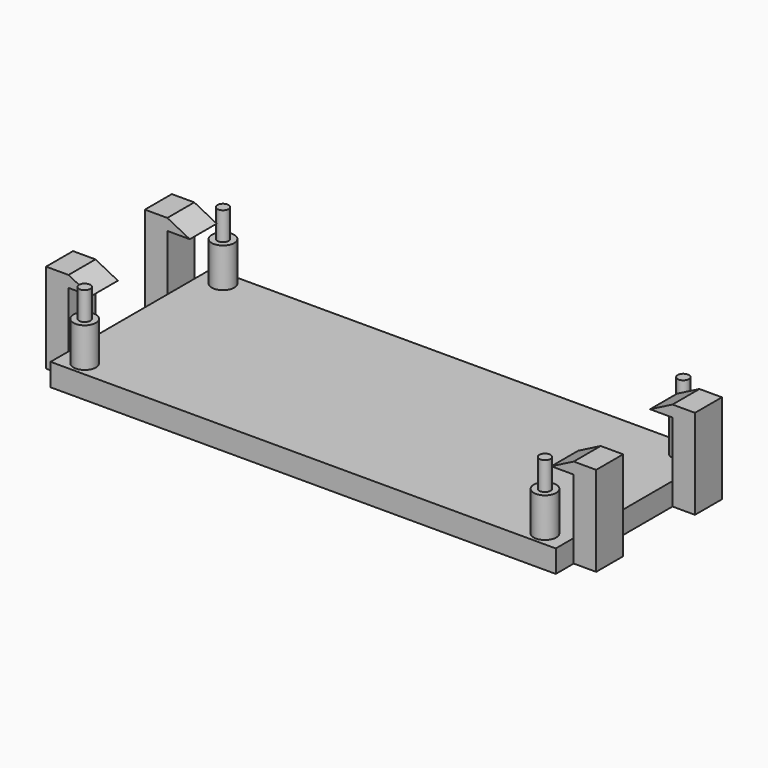
from build123d import *

# Parameters (mm, degrees)
F0_R     = 1
F0_R_2   = 0.5
F1_DEPTH = 2
F2_DEPTH = 5.5
F3_DEPTH = 8
F0_W     = 2
F0_H     = 3
F4_DEPTH = 8
F6_DEPTH = 3


# Not quite as in the source:
# - a feature names something its author has since deleted; it is built from what else it names


with BuildPart() as f1:
    # F0 (on Top) → F1 (new body)
    with BuildSketch(Plane.XY):
        Polygon((22.5, 9), (-22.5, 9), (-22.5, 7), (-22.5, 4), (-22.5, -4), (-22.5, -7), (-22.5, -9), (22.5, -9), (22.5, -7), (22.5, -4), (22.5, 4), (22.5, 7), align=None)
        with Locations((-20.5, -7.7)):
            Circle(F0_R, mode=Mode.SUBTRACT)
        with Locations((20.5, -7.7)):
            Circle(F0_R, mode=Mode.SUBTRACT)
        with Locations((-20.5, 7.7)):
            Circle(F0_R, mode=Mode.SUBTRACT)
        with Locations((20.5, 7.7)):
            Circle(F0_R, mode=Mode.SUBTRACT)
        with Locations((-20.5, 7.7)):
            Circle(F0_R)
        with Locations((-20.5, 7.7)):
            Circle(F0_R_2, mode=Mode.SUBTRACT)
        with Locations((20.5, 7.7)):
            Circle(F0_R)
        with Locations((20.5, 7.7)):
            Circle(F0_R_2, mode=Mode.SUBTRACT)
        with Locations((20.5, -7.7)):
            Circle(F0_R)
        with Locations((20.5, -7.7)):
            Circle(F0_R_2, mode=Mode.SUBTRACT)
        with Locations((-20.5, -7.7)):
            Circle(F0_R)
        with Locations((-20.5, -7.7)):
            Circle(F0_R_2, mode=Mode.SUBTRACT)
        with Locations((-20.5, 7.7)):
            Circle(F0_R_2)
        with Locations((20.5, 7.7)):
            Circle(F0_R_2)
        with Locations((20.5, -7.7)):
            Circle(F0_R_2)
        with Locations((-20.5, -7.7)):
            Circle(F0_R_2)
    extrude(amount=F1_DEPTH)

    # F0 (on Top) → F2 (join)
    with BuildSketch(Plane.XY):
        with Locations((-20.5, 7.7)):
            Circle(F0_R)
        with Locations((-20.5, 7.7)):
            Circle(F0_R_2, mode=Mode.SUBTRACT)
        with Locations((-20.5, 7.7)):
            Circle(F0_R_2)
        with Locations((-20.5, -7.7)):
            Circle(F0_R)
        with Locations((-20.5, -7.7)):
            Circle(F0_R_2, mode=Mode.SUBTRACT)
        with Locations((-20.5, -7.7)):
            Circle(F0_R_2)
        with Locations((20.5, 7.7)):
            Circle(F0_R)
        with Locations((20.5, 7.7)):
            Circle(F0_R_2, mode=Mode.SUBTRACT)
        with Locations((20.5, 7.7)):
            Circle(F0_R_2)
        with Locations((20.5, -7.7)):
            Circle(F0_R)
        with Locations((20.5, -7.7)):
            Circle(F0_R_2, mode=Mode.SUBTRACT)
        with Locations((20.5, -7.7)):
            Circle(F0_R_2)
    extrude(amount=F2_DEPTH)

    # F0 (on Top) → F3 (join)
    with BuildSketch(Plane.XY):
        with Locations((-20.5, 7.7)):
            Circle(F0_R_2)
        with Locations((20.5, 7.7)):
            Circle(F0_R_2)
        with Locations((20.5, -7.7)):
            Circle(F0_R_2)
        with Locations((-20.5, -7.7)):
            Circle(F0_R_2)
    extrude(amount=F3_DEPTH)

    # F0 (on Top) → F4 (join)
    with BuildSketch(Plane.XY):
        with Locations((-23.5, 5.5)):
            Rectangle(F0_W, F0_H)
    extrude(amount=F4_DEPTH)

    # F5 (on face) → F6 (join, through all)
    with BuildSketch(Plane.XZ.offset(-4)):
        Polygon((-22.5, 8), (-22.5, 6.980669219), (-20.5, 6.980669219), align=None)
    extrude(amount=-F6_DEPTH)

    # F7: F1 across plane


with BuildPart() as f1_1:
    add(f1.part)
    add(f1.part.mirror(Plane.XZ))

    # F8: F1 across plane


with BuildPart() as f1_2:
    add(f1_1.part)
    add(f1_1.part.mirror(Plane.YZ))


solid = f1_2.part
